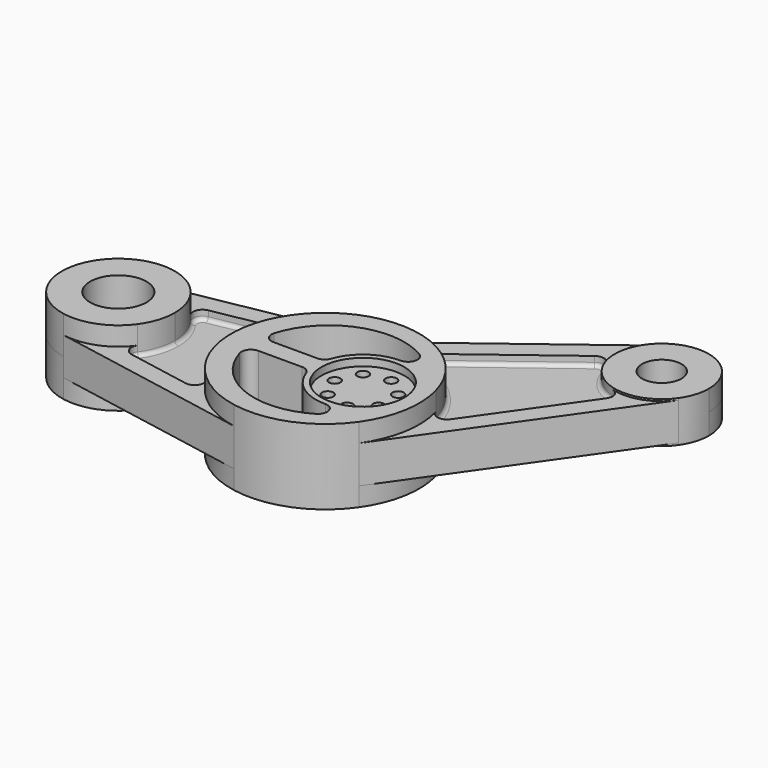
from build123d import *

# Parameters (mm, degrees)
F0_R     = 15
F1_DEPTH = 20
F0_R_2   = 22
F2_DEPTH = 10
F3_DEPTH = 5
F0_R_3   = 3
F4_DEPTH = 16
F0_R_4   = 10.5
F5_DEPTH = 11
F6_R     = 2


with BuildPart() as f1:
    # F0 (on Top) → F1 (new body, symmetric)
    with BuildSketch(Plane.XY):
        with BuildLine():
            ThreePointArc((-105.6842108418, 17.5710670597), (-118.8415377441, 27.8475981026), (-135.4545454545, 29.4999649811))
            ThreePointArc((-135.4545454545, 29.4999649811), (-160, 0), (-135.4545454545, -29.4999649811))
            ThreePointArc((-135.4545454545, -29.4999649811), (-118.8415377441, -27.8475981026), (-105.6842108418, -17.5710670597))
            ThreePointArc((-105.6842108418, -17.5710670597), (-101.4564046173, -9.233805425), (-100, 0))
            ThreePointArc((-100, 0), (-101.4564046173, 9.233805425), (-105.6842108418, 17.5710670597))
        make_face()
        with Locations((-130, 0)):
            Circle(F0_R, mode=Mode.SUBTRACT)
    extrude(amount=F1_DEPTH, both=True)



with BuildPart() as f1b:
    # F0 (on Top) → F1, piece 2 (new body, symmetric)
    with BuildSketch(Plane.XY):
        with BuildLine():
            ThreePointArc((-29.0909090909, -49.1666083018), (-1.0982935918, -46.2895830059), (20.9072911046, -28.7505397251))
            ThreePointArc((20.9072911046, -28.7505397251), (27.6726575472, -15.0770594741), (30, 0))
            ThreePointArc((30, 0), (29.5504209908, 6.6899760564), (28.2097688146, 13.2596452005))
            ThreePointArc((28.2097688146, 13.2596452005), (17.273093336, 33.3274138386), (-1.4510675533, 46.4320697911))
            ThreePointArc((-1.4510675533, 46.4320697911), (-15.0772998602, 49.7570801327), (-29.0909090909, 49.1666083018))
            ThreePointArc((-29.0909090909, 49.1666083018), (-49.1877488917, 40.5964938712), (-63.7117153904, 24.2752124117))
            ThreePointArc((-63.7117153904, 24.2752124117), (-70, 0), (-63.7117153904, -24.2752124117))
            ThreePointArc((-63.7117153904, -24.2752124117), (-49.1877488917, -40.5964938712), (-29.0909090909, -49.1666083018))
        make_face()
        with BuildLine():
            Line((-51.5410196625, -5), (-28.2842712475, -5))
            ThreePointArc((-28.2842712475, -5), (-25.3975199015, -5.9175170954), (-23.5702260396, -8.3333333333))
            ThreePointArc((-23.5702260396, -8.3333333333), (-14.42430499, -20.4190946311), (0.0231481481, -24.9999892833))
            ThreePointArc((0.0231481481, -24.9999892833), (4.845278682, -28.6614487437), (2.6031746032, -34.2856995885))
            ThreePointArc((2.6031746032, -34.2856995885), (-32.4635802649, -37.2934960271), (-56.3325939, -11.4285714286))
            ThreePointArc((-56.3325939, -11.4285714286), (-55.5499382912, -7.0119284767), (-51.5410196625, -5))
        make_face(mode=Mode.SUBTRACT)
        Circle(F0_R_2, mode=Mode.SUBTRACT)
        with BuildLine():
            ThreePointArc((2.6031746032, 34.2856995885), (4.845278682, 28.6614487437), (0.0231481481, 24.9999892833))
            ThreePointArc((0.0231481481, 24.9999892833), (-14.42430499, 20.4190946311), (-23.5702260396, 8.3333333333))
            ThreePointArc((-23.5702260396, 8.3333333333), (-25.3975199015, 5.9175170954), (-28.2842712475, 5))
            Line((-28.2842712475, 5), (-51.5410196625, 5))
            ThreePointArc((-51.5410196625, 5), (-55.5499382912, 7.0119284767), (-56.3325939, 11.4285714286))
            ThreePointArc((-56.3325939, 11.4285714286), (-32.4635802649, 37.2934960271), (2.6031746032, 34.2856995885))
        make_face(mode=Mode.SUBTRACT)
    extrude(amount=F1_DEPTH, both=True)


with BuildPart() as f1_1:
    add(f1.part)

    add(f1b.part)  # F2 merges F1b
    # F0 (on Top) → F2 (join, symmetric)
    with BuildSketch(Plane.XY):
        with BuildLine():
            ThreePointArc((-63.7117153904, 24.2752124117), (-49.1877488917, 40.5964938712), (-29.0909090909, 49.1666083018))
            Line((-29.0909090909, 49.1666083018), (-135.4545454545, 29.4999649811))
            ThreePointArc((-135.4545454545, 29.4999649811), (-118.8415377441, 27.8475981026), (-105.6842108418, 17.5710670597))
            ThreePointArc((-105.6842108418, 17.5710670597), (-106.2728456659, 22.3593219456), (-102.5406702246, 25.4162390665))
            Line((-102.5406702246, 25.4162390665), (-68.9919778385, 31.619394483))
            ThreePointArc((-68.9919778385, 31.619394483), (-64.0232375423, 29.621508542), (-63.7117153904, 24.2752124117))
        make_face()
        with BuildLine():
            Line((-135.4545454545, -29.4999649811), (-29.0909090909, -49.1666083018))
            ThreePointArc((-29.0909090909, -49.1666083018), (-49.1877488917, -40.5964938712), (-63.7117153904, -24.2752124117))
            ThreePointArc((-63.7117153904, -24.2752124117), (-64.0232375423, -29.621508542), (-68.9919778385, -31.619394483))
            Line((-68.9919778385, -31.619394483), (-102.5406702246, -25.4162390665))
            ThreePointArc((-102.5406702246, -25.4162390665), (-106.2728456659, -22.3593219456), (-105.6842108418, -17.5710670597))
            ThreePointArc((-105.6842108418, -17.5710670597), (-118.8415377441, -27.8475981026), (-135.4545454545, -29.4999649811))
        make_face()
        with BuildLine():
            ThreePointArc((56.0990159053, 91.1222535905), (56.0973330219, 106.2675258234), (64.840085954, 118.634560432))
            Line((64.840085954, 118.634560432), (-24.0325974922, 51.3968230973))
            ThreePointArc((-24.0325974922, 51.3968230973), (-26.4315765459, 49.9864640746), (-29.0909090909, 49.1666083018))
            ThreePointArc((-29.0909090909, 49.1666083018), (-15.0772998602, 49.7570801327), (-1.4510675533, 46.4320697911))
            ThreePointArc((-1.4510675533, 46.4320697911), (-4.5514765242, 50.4082085938), (-2.6128950505, 55.0626814356))
            Line((-2.6128950505, 55.0626814356), (48.3173604119, 93.594601553))
            ThreePointArc((48.3173604119, 93.594601553), (52.8480788974, 94.3724682159), (56.0990159053, 91.1222535905))
        make_face()
        with BuildLine():
            Line((20.9072911046, -28.7505397251), (100.3773352156, 84.3222672425))
            ThreePointArc((100.3773352156, 84.3222672425), (88.3244553995, 75.1512606468), (73.1884371125, 74.6218985242))
            ThreePointArc((73.1884371125, 74.6218985242), (76.550641894, 71.4869239552), (75.9321157128, 66.9317168355))
            Line((75.9321157128, 66.9317168355), (37.1214748065, 11.710555748))
            ThreePointArc((37.1214748065, 11.710555748), (32.1744542827, 9.6594788843), (28.2097688146, 13.2596452005))
            ThreePointArc((28.2097688146, 13.2596452005), (29.5504209908, 6.6899760564), (30, 0))
            ThreePointArc((30, 0), (27.6726575472, -15.0770594741), (20.9072911046, -28.7505397251))
        make_face()
    extrude(amount=F2_DEPTH, both=True)

    # F0 (on Top) → F3 (join, symmetric)
    with BuildSketch(Plane.XY):
        with BuildLine():
            ThreePointArc((-63.7117153904, -24.2752124117), (-70, 0), (-63.7117153904, 24.2752124117))
            ThreePointArc((-63.7117153904, 24.2752124117), (-64.0232375423, 29.621508542), (-68.9919778385, 31.619394483))
            Line((-68.9919778385, 31.619394483), (-102.5406702246, 25.4162390665))
            ThreePointArc((-102.5406702246, 25.4162390665), (-106.2728456659, 22.3593219456), (-105.6842108418, 17.5710670597))
            ThreePointArc((-105.6842108418, 17.5710670597), (-101.4564046173, 9.233805425), (-100, 0))
            ThreePointArc((-100, 0), (-101.4564046173, -9.233805425), (-105.6842108418, -17.5710670597))
            ThreePointArc((-105.6842108418, -17.5710670597), (-106.2728456659, -22.3593219456), (-102.5406702246, -25.4162390665))
            Line((-102.5406702246, -25.4162390665), (-68.9919778385, -31.619394483))
            ThreePointArc((-68.9919778385, -31.619394483), (-64.0232375423, -29.621508542), (-63.7117153904, -24.2752124117))
        make_face()
        with BuildLine():
            ThreePointArc((73.1884371125, 74.6218985242), (62.5587046841, 80.7126185155), (56.0990159053, 91.1222535905))
            ThreePointArc((56.0990159053, 91.1222535905), (52.8480788974, 94.3724682159), (48.3173604119, 93.594601553))
            Line((48.3173604119, 93.594601553), (-2.6128950505, 55.0626814356))
            ThreePointArc((-2.6128950505, 55.0626814356), (-4.5514765242, 50.4082085938), (-1.4510675533, 46.4320697911))
            ThreePointArc((-1.4510675533, 46.4320697911), (17.273093336, 33.3274138386), (28.2097688146, 13.2596452005))
            ThreePointArc((28.2097688146, 13.2596452005), (32.1744542827, 9.6594788843), (37.1214748065, 11.710555748))
            Line((37.1214748065, 11.710555748), (75.9321157128, 66.9317168355))
            ThreePointArc((75.9321157128, 66.9317168355), (76.550641894, 71.4869239552), (73.1884371125, 74.6218985242))
        make_face()
    extrude(amount=F3_DEPTH, both=True)

    # F0 (on Top) → F4 (join, symmetric)
    with BuildSketch(Plane.XY):
        Circle(F0_R_2)
        with Locations((3.3378140093, -14.6239186827)):
            Circle(F0_R_3, mode=Mode.SUBTRACT)
        with Locations((-9.3523470279, -11.727472237)):
            Circle(F0_R_3, mode=Mode.SUBTRACT)
        with Locations((-15, 0)):
            Circle(F0_R_3, mode=Mode.SUBTRACT)
        with Locations((-9.3523470279, 11.727472237)):
            Circle(F0_R_3, mode=Mode.SUBTRACT)
        with Locations((3.3378140093, 14.6239186827)):
            Circle(F0_R_3, mode=Mode.SUBTRACT)
        with Locations((13.5145330185, -6.5082560868)):
            Circle(F0_R_3, mode=Mode.SUBTRACT)
        with Locations((13.5145330185, 6.5082560868)):
            Circle(F0_R_3, mode=Mode.SUBTRACT)
    extrude(amount=F4_DEPTH, both=True)

    # F0 (on Top) → F5 (join, symmetric)
    with BuildSketch(Plane.XY):
        with BuildLine():
            ThreePointArc((100.3773352156, 84.3222672425), (103.7600184369, 91.159007368), (104.9236896633, 98.697537105))
            ThreePointArc((104.9236896633, 98.697537105), (91.0571955637, 121.0815726297), (64.840085954, 118.634560432))
            ThreePointArc((64.840085954, 118.634560432), (56.0973330219, 106.2675258234), (56.0990159053, 91.1222535905))
            ThreePointArc((56.0990159053, 91.1222535905), (62.5587046841, 80.7126185155), (73.1884371125, 74.6218985242))
            ThreePointArc((73.1884371125, 74.6218985242), (88.3244553995, 75.1512606468), (100.3773352156, 84.3222672425))
        make_face()
        with Locations((79.9236896633, 98.697537105)):
            Circle(F0_R_4, mode=Mode.SUBTRACT)
    extrude(amount=F5_DEPTH, both=True)

    # F6
    f6_edges = [f1_1.edges().sort_by_distance(p)[0] for p in [
        (-85.766324, 28.517817, 5),
        (22.852233, 74.328641, 5),
        (56.526795, 39.321136, -5),
        (-85.766324, -28.517817, -5),
        (-70, 0, -5),
        (17.273093, 33.327414, -5),
        (-64.023238, -29.621509, -5),
        (-106.272846, -22.359322, -5),
        (-64.023238, -29.621509, 5),
        (-85.766324, -28.517817, 5),
        (-106.272846, -22.359322, 5),
        (-64.023238, 29.621509, -5),
        (-85.766324, 28.517817, -5),
        (-106.272846, 22.359322, -5),
        (-101.456405, 9.233805, -5),
        (-101.456405, -9.233805, -5),
        (76.550642, 71.486924, -5),
        (32.174454, 9.659479, -5),
        (76.550642, 71.486924, 5),
        (56.526795, 39.321136, 5),
        (32.174454, 9.659479, 5),
        (-70, 0, 5),
        (17.273093, 33.327414, 5),
        (62.558705, 80.712619, -5),
        (52.848079, 94.372468, -5),
        (22.852233, 74.328641, -5),
        (-4.551477, 50.408209, -5),
        (-101.456405, 9.233805, 5),
        (-101.456405, -9.233805, 5),
        (-64.023238, 29.621509, 5),
        (-106.272846, 22.359322, 5),
        (62.558705, 80.712619, 5),
        (52.848079, 94.372468, 5),
        (-4.551477, 50.408209, 5),
    ]]
    fillet(f6_edges, radius=F6_R)


solid = f1_1.part
